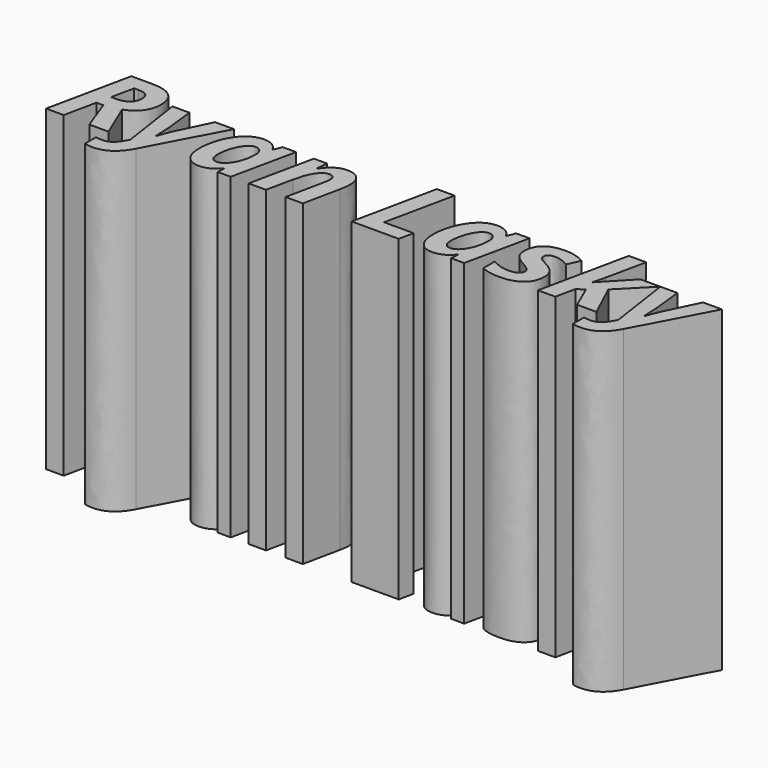
from build123d import *

# Parameters (mm, degrees)
F0_TEXT_SIZE = 1.8604651163
F1_DEPTH     = 5


# Not quite as in the source:
# - Text() gives the source's letters only with a copy of the font that has no kerning and outlines rounded to 1/6400 em; it was checked with that copy


with BuildPart() as f1:
    # F0 (on Top) → F1 (new body)
    with BuildSketch(Plane.XY):
        with Locations((-1.0013464183, -0.6829865684)):
            Text('Ryan Lasky', F0_TEXT_SIZE, font='Open Sans', font_style=FontStyle.BOLDITALIC, text_align=(TextAlign.LEFT, TextAlign.BOTTOM))
    extrude(amount=F1_DEPTH)


solid = f1.part
